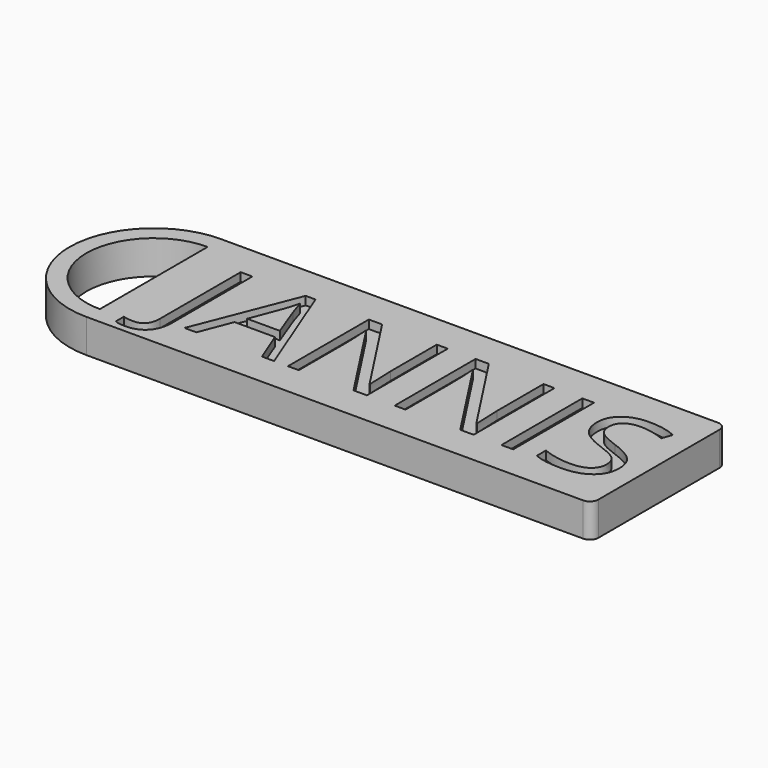
from build123d import *

# Parameters (mm, degrees)
F4_DEPTH     = 2
F1_R         = 0.5
F2_TEXT_SIZE = 8.4076194051
F3_DEPTH     = 0.5


# Not quite as in the source:
# - Text() gives the source's letters only with a copy of the font that has no kerning and outlines rounded to 1/6400 em; it was checked with that copy


with BuildPart() as f4:
    # F0 (on Top) → F4 (new body)
    with BuildSketch(Plane.XY):
        Polygon((24.7291392038, 3.2207785361), (-5.2708607962, 3.2207785361), (-5.2708607962, 2.2207785361), (-5.2708607962, -5.7792214639), (-5.2708607962, -6.7792214639), (24.7291392038, -6.7792214639), align=None)
        with BuildLine():
            Line((-5.2708607962, 2.2207785361), (-5.2708607962, 3.2207785361))
            ThreePointArc((-5.2708607962, 3.2207785361), (-10.2708607962, -1.7792214639), (-5.2708607962, -6.7792214639))
            Line((-5.2708607962, -6.7792214639), (-5.2708607962, -5.7792214639))
            ThreePointArc((-5.2708607962, -5.7792214639), (-9.2708607962, -1.7792214639), (-5.2708607962, 2.2207785361))
        make_face()
    extrude(amount=F4_DEPTH)

    # F1
    f1_edges = [f4.edges().sort_by_distance(p)[0] for p in [
        (24.729139, -6.779221, 1),
        (24.729139, 3.220779, 1),
    ]]
    fillet(f1_edges, radius=F1_R)

    # F2 (on face) → F3 (cut)
    with BuildSketch(Plane.XY.offset(2)):
        with Locations((-3.2708607962, -4.8059644498)):
            Text('JANNIS', F2_TEXT_SIZE, font='Open Sans', text_align=(TextAlign.LEFT, TextAlign.BOTTOM))
    extrude(amount=-F3_DEPTH, mode=Mode.SUBTRACT)


solid = f4.part
